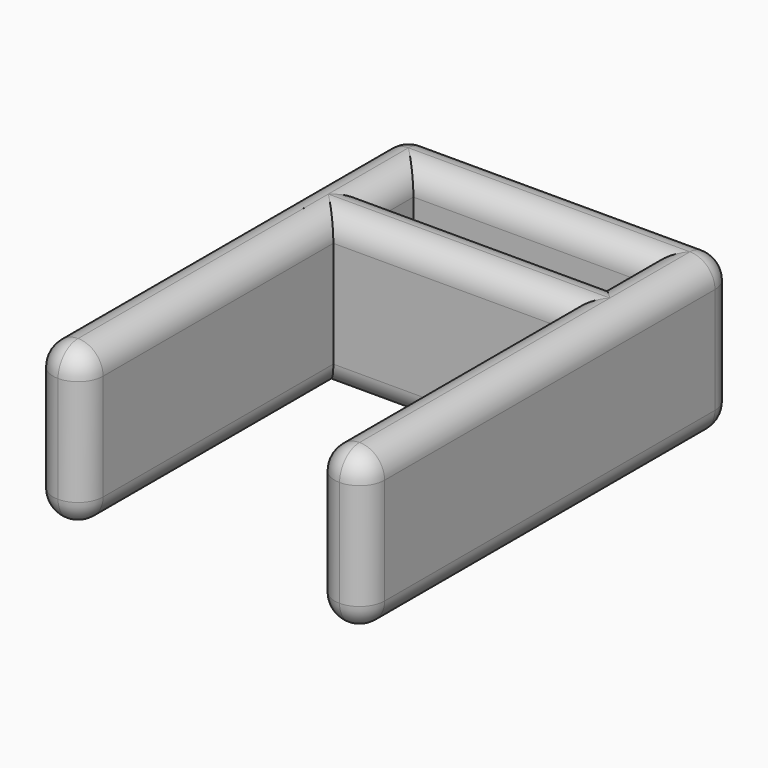
from build123d import *

# Parameters (mm, degrees)
F1_DEPTH = 25
F2_R     = 3.99999


# Not quite as in the source:
# - a fillet or chamfer is up to 0.001 mm smaller than in the source, because OpenCascade refuses the exact size


with BuildPart() as f1:
    # F0 (on Top) → F1 (new body)
    with BuildSketch(Plane.XY):
        Polygon((18.5, 25), (18.5, -25), (26.5, -25), (26.5, 33), (18.5, 33), (-18.5, 33), (-26.5, 33), (-26.5, -25), (-18.5, -25), (-18.5, 25), align=None)
        Polygon((18.5, 33), (26.5, 33), (26.5, 49), (-26.5, 49), (-26.5, 33), (-18.5, 33), (-18.5, 41), (18.5, 41), align=None)
    extrude(amount=F1_DEPTH)

    # F2 (radius 4 in the source; OpenCascade refuses exactly that, so slightly less here)
    f2_edges = [f1.edges().sort_by_distance(p)[0] for p in [
        (-26.5, 49, 12.5),
        (26.5, 49, 12.5),
        (-18.5, -25, 12.5),
        (18.5, -25, 12.5),
        (-26.5, -25, 12.5),
        (26.5, -25, 12.5),
        (0, 33, 25),
        (-18.5, 37, 25),
        (0, 41, 25),
        (18.5, 37, 25),
        (-18.5, 0, 25),
        (0, 25, 25),
        (26.5, 12, 0),
        (26.5, 12, 25),
        (18.5, 0, 0),
        (22.5, -25, 0),
        (0, 49, 0),
        (-26.5, 12, 0),
        (-22.5, -25, 0),
        (-18.5, 0, 0),
        (0, 25, 0),
        (0, 33, 0),
        (-18.5, 37, 0),
        (0, 41, 0),
        (18.5, 37, 0),
        (18.5, 0, 25),
        (22.5, -25, 25),
        (0, 49, 25),
        (-26.5, 12, 25),
        (-22.5, -25, 25),
    ]]
    fillet(f2_edges, radius=F2_R)


solid = f1.part
